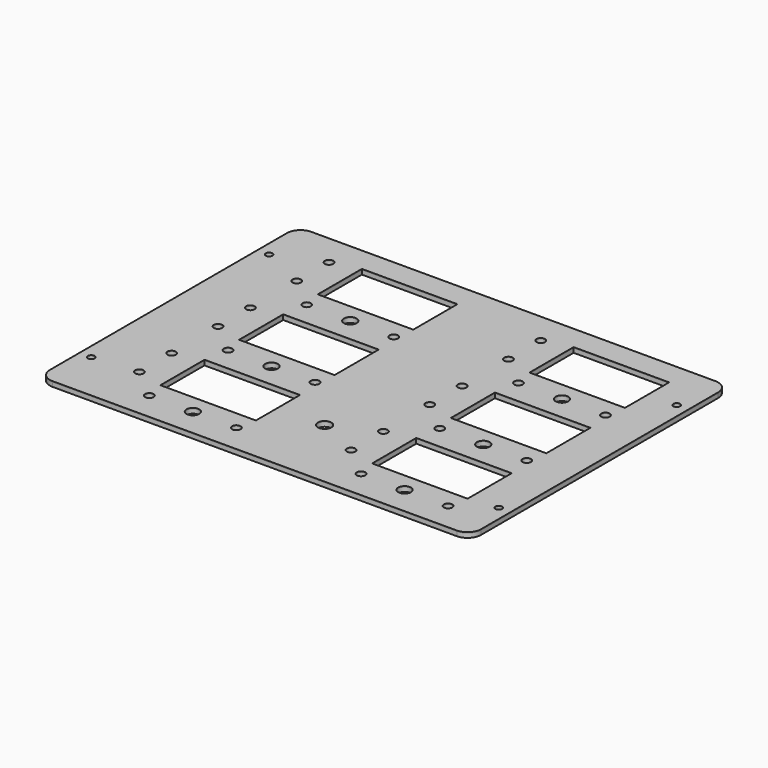
from build123d import *

# Parameters (mm, degrees)
F3_DEPTH  = 0.396875
F5_DEPTH  = 1.984375
F6_W      = 45
F6_H      = 26
F7_DEPTH  = 2.38125
F8_R      = 3.175
F8_R_2    = 2
F10_DEPTH = 2.38125
F9_R      = 3
F11_DEPTH = 2.38125
F12_R     = 1.5875
F13_DEPTH = 2.38125


# Not quite as in the source:
# - a length typed as a fraction of an inch, garbled in the dataset ("3 / 203.2 mm" for 3/8 in), is restored


with BuildPart() as f3:
    # F0 (on Top) → F3 (new body)
    with BuildSketch(Plane.XY):
        with BuildLine():
            ThreePointArc((0, 6.35), (1.8598719395, 1.8598719395), (6.35, 0))
            Line((6.35, 0), (196.85, 0))
            ThreePointArc((196.85, 0), (201.3401280605, 1.8598719395), (203.2, 6.35))
            Line((203.2, 6.35), (203.2, 146.05))
            ThreePointArc((203.2, 146.05), (201.3401280605, 150.5401280605), (196.85, 152.4))
            Line((196.85, 152.4), (6.35, 152.4))
            ThreePointArc((6.35, 152.4), (1.8598719395, 150.5401280605), (0, 146.05))
            Line((0, 146.05), (0, 6.35))
        make_face()
    extrude(amount=-F3_DEPTH)


with BuildPart() as f5:
    # F4 (on face) → F5 (new body)
    with BuildSketch(Plane(origin=(0, 0, -0.396875), x_dir=(1, 0, 0), z_dir=(0, 0, -1))):
        with BuildLine():
            Line((6.35, -152.4), (196.85, -152.4))
            ThreePointArc((196.85, -152.4), (201.3401280605, -150.5401280605), (203.2, -146.05))
            Line((203.2, -146.05), (203.2, -6.35))
            ThreePointArc((203.2, -6.35), (201.3401280605, -1.8598719395), (196.85, 0))
            Line((196.85, 0), (6.35, 0))
            ThreePointArc((6.35, 0), (1.8598719395, -1.8598719395), (0, -6.35))
            Line((0, -6.35), (0, -146.05))
            ThreePointArc((0, -146.05), (1.8598719395, -150.5401280605), (6.35, -152.4))
        make_face()
    extrude(amount=F5_DEPTH)


with BuildPart() as f7_tool:
    # F6 (on face) → F7 (new body)
    with BuildSketch(Plane.XY):
        with Locations((161.65, 127.97)):
            Rectangle(F6_W, F6_H)
        with Locations((161.65, 81.615)):
            Rectangle(F6_W, F6_H)
        with Locations((161.65, 35.26)):
            Rectangle(F6_W, F6_H)
        with Locations((61.87, 127.97)):
            Rectangle(F6_W, F6_H)
        with Locations((61.87, 81.615)):
            Rectangle(F6_W, F6_H)
        with Locations((61.87, 35.26)):
            Rectangle(F6_W, F6_H)
    extrude(amount=-F7_DEPTH)


with BuildPart() as f3_1:
    add(f3.part)

    # F7: cut by f7_tool
    add(f7_tool.part, mode=Mode.SUBTRACT)


with BuildPart() as f5_1:
    add(f5.part)

    # F7: cut by f7_tool
    add(f7_tool.part, mode=Mode.SUBTRACT)


with BuildPart() as f10_tool:
    # F8 (on face) → F10 (new body)
    with BuildSketch(Plane.XY):
        with Locations((106.3625, 35.26)):
            Circle(F8_R)
        with Locations((126.45, 137.495)):
            Circle(F8_R_2)
        with Locations((141.15, 105.97)):
            Circle(F8_R_2)
        with Locations((182.15, 105.97)):
            Circle(F8_R_2)
        with Locations((126.45, 118.445)):
            Circle(F8_R_2)
        with Locations((182.15, 59.615)):
            Circle(F8_R_2)
        with Locations((141.15, 59.615)):
            Circle(F8_R_2)
        with Locations((126.45, 91.14)):
            Circle(F8_R_2)
        with Locations((126.45, 72.09)):
            Circle(F8_R_2)
        with Locations((182.15, 13.26)):
            Circle(F8_R_2)
        with Locations((141.15, 13.26)):
            Circle(F8_R_2)
        with Locations((126.45, 44.785)):
            Circle(F8_R_2)
        with Locations((126.45, 25.735)):
            Circle(F8_R_2)
        with Locations((82.37, 105.97)):
            Circle(F8_R_2)
        with Locations((41.37, 105.97)):
            Circle(F8_R_2)
        with Locations((26.67, 137.495)):
            Circle(F8_R_2)
        with Locations((26.67, 118.445)):
            Circle(F8_R_2)
        with Locations((82.37, 59.615)):
            Circle(F8_R_2)
        with Locations((41.37, 59.615)):
            Circle(F8_R_2)
        with Locations((26.67, 91.14)):
            Circle(F8_R_2)
        with Locations((26.67, 72.09)):
            Circle(F8_R_2)
        with Locations((82.37, 13.26)):
            Circle(F8_R_2)
        with Locations((41.37, 13.26)):
            Circle(F8_R_2)
        with Locations((26.67, 44.785)):
            Circle(F8_R_2)
        with Locations((26.67, 25.735)):
            Circle(F8_R_2)
    extrude(amount=-F10_DEPTH)


with BuildPart() as f3_2:
    add(f3_1.part)

    # F10: cut by f10_tool
    add(f10_tool.part, mode=Mode.SUBTRACT)


with BuildPart() as f5_2:
    add(f5_1.part)

    # F10: cut by f10_tool
    add(f10_tool.part, mode=Mode.SUBTRACT)


with BuildPart() as f11_tool:
    # F9 (on face) → F11 (new body)
    with BuildSketch(Plane.XY):
        with Locations((161.65, 105.9784)):
            Circle(F9_R)
        with Locations((161.65, 59.6234)):
            Circle(F9_R)
        with Locations((161.65, 13.2684)):
            Circle(F9_R)
        with Locations((61.87, 105.9784)):
            Circle(F9_R)
        with Locations((61.87, 59.6234)):
            Circle(F9_R)
        with Locations((61.87, 13.2684)):
            Circle(F9_R)
    extrude(amount=-F11_DEPTH)


with BuildPart() as f3_3:
    add(f3_2.part)

    # F11: cut by f11_tool
    add(f11_tool.part, mode=Mode.SUBTRACT)


with BuildPart() as f5_3:
    add(f5_2.part)

    # F11: cut by f11_tool
    add(f11_tool.part, mode=Mode.SUBTRACT)


with BuildPart() as f13_tool:
    # F12 (on face) → F13 (new body)
    with BuildSketch(Plane.XY):
        with Locations((5.5499, 128.5875)):
            Circle(F12_R)
        with Locations((5.5499, 23.8125)):
            Circle(F12_R)
        with Locations((197.6374, 128.5875)):
            Circle(F12_R)
        with Locations((197.6374, 23.8125)):
            Circle(F12_R)
    extrude(amount=-F13_DEPTH)


with BuildPart() as f3_4:
    add(f3_3.part)

    # F13: cut by f13_tool
    add(f13_tool.part, mode=Mode.SUBTRACT)


with BuildPart() as f5_4:
    add(f5_3.part)

    # F13: cut by f13_tool
    add(f13_tool.part, mode=Mode.SUBTRACT)


solid = Compound([f3_4.part, f5_4.part])
